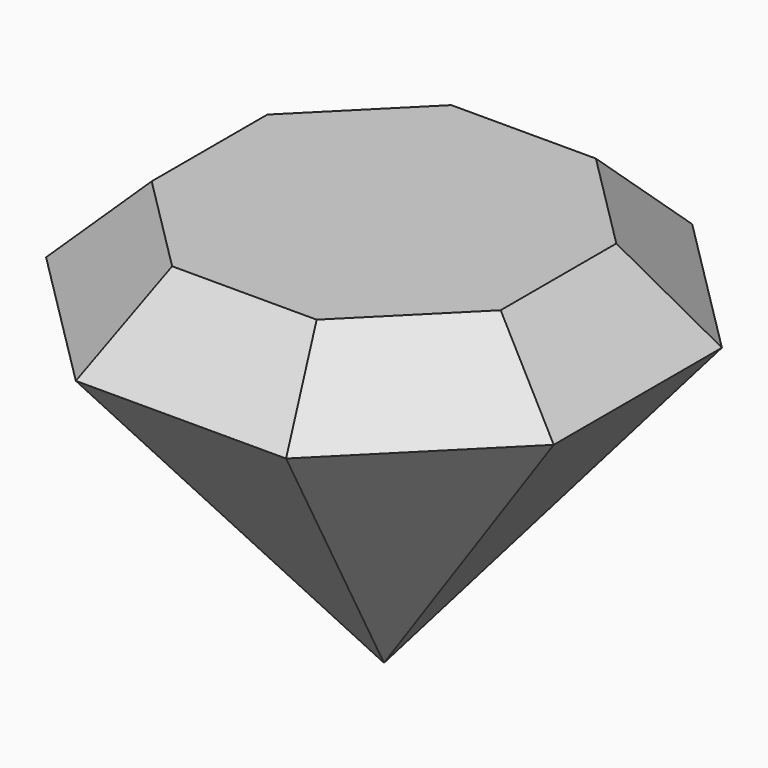
from build123d import *

# Parameters (mm, degrees)
F1_DEPTH = 0.5
F2_SIZE2 = 0.49999
F2_SIZE  = 0.49999


# Not quite as in the source:
# - a fillet or chamfer is up to 0.001 mm smaller than in the source, because OpenCascade refuses the exact size


with BuildPart() as f1:
    # F0 (on Top) → F1 (new body)
    with BuildSketch(Plane.XY):
        Polygon((-1.6, 0.6627416998), (-1.6, -0.6627416998), (-0.6627416998, -1.6), (0.6627416998, -1.6), (1.6, -0.6627416998), (1.6, 0.6627416998), (0.6627416998, 1.6), (-0.6627416998, 1.6), align=None)
    extrude(amount=F1_DEPTH)

    # F2 (size 0.5 and 0.5 in the source; OpenCascade refuses exactly that, so slightly less here)
    f2_edges = [f1.edges().sort_by_distance(p)[0] for p in [
        (-1.131371, 1.131371, 0.5),
        (-1.6, 0, 0.5),
        (-1.131371, -1.131371, 0.5),
        (0, -1.6, 0.5),
        (1.131371, -1.131371, 0.5),
        (1.6, 0, 0.5),
        (1.131371, 1.131371, 0.5),
        (0, 1.6, 0.5),
    ]]
    chamfer(f2_edges, length=F2_SIZE, length2=F2_SIZE2)

    # F1_face (on face) → F5 section 0
    with BuildSketch(Plane(origin=(0, 0, 0), x_dir=(1, 0, 0), z_dir=(0, 0, -1)), mode=Mode.PRIVATE) as f5_s0:
        Polygon((-1.6, -0.6627416998), (-0.6627416998, -1.6), (0.6627416998, -1.6), (1.6, -0.6627416998), (1.6, 0.6627416998), (0.6627416998, 1.6), (-0.6627416998, 1.6), (-1.6, 0.6627416998), align=None)
    loft([f5_s0.sketch, Vertex(0, 0, -2)])


solid = f1.part
